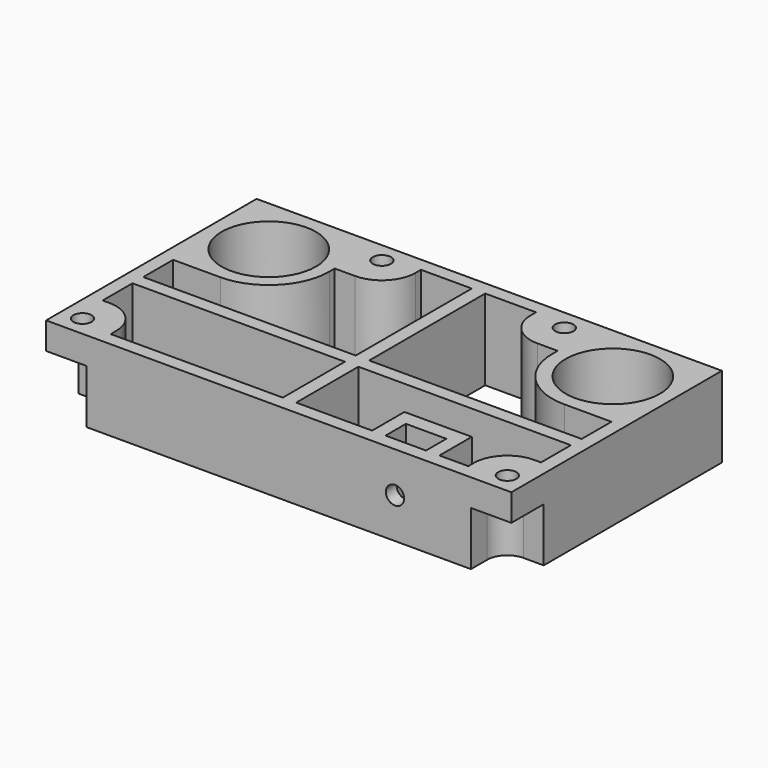
from build123d import *

# Parameters (mm, degrees)
F0_W      = 109.6809846
F0_H      = 62.036204
F0_R      = 2.15265
F0_W_2    = 9.525
F0_H_2    = 6
F0_R_2    = 11.1125
F1_DEPTH  = 19.05
F2_W      = 9.525
F2_H      = 9.525
F3_DEPTH  = 12.7
F4_R      = 4.76249
F6_DEPTH  = 19.05
F7_R      = 2.15265
F8_DEPTH  = 3.175
F9_R      = 1.7272
F10_DEPTH = 3.525


# Not quite as in the source:
# - a fillet or chamfer is up to 0.001 mm smaller than in the source, because OpenCascade refuses the exact size


with BuildPart() as f1:
    # F0 (on Top) → F1 (new body)
    with BuildSketch(Plane.XY):
        with Locations((0, -16.730602)):
            Rectangle(F0_W, F0_H)
        with Locations((-50.0779923, -42.986204)):
            Circle(F0_R, mode=Mode.SUBTRACT)
        with Locations((27.406219, -41.573704)):
            Rectangle(F0_W_2, F0_H_2, mode=Mode.SUBTRACT)
        with Locations((50.0779923, -42.986204)):
            Circle(F0_R, mode=Mode.SUBTRACT)
        with Locations((-40.5529923, 0)):
            Circle(F0_R_2, mode=Mode.SUBTRACT)
        with Locations((-21.5029923, 9.525)):
            Circle(F0_R, mode=Mode.SUBTRACT)
        with Locations((21.5029923, 9.525)):
            Circle(F0_R, mode=Mode.SUBTRACT)
        with Locations((40.5529923, 0)):
            Circle(F0_R_2, mode=Mode.SUBTRACT)
    extrude(amount=F1_DEPTH)

    # F2 (on face) → F3 (cut)
    with BuildSketch(Plane(origin=(0, 0, 0), x_dir=(1, 0, 0), z_dir=(0, 0, -1))):
        with Locations((-21.5029923, -9.525)):
            Rectangle(F2_W, F2_H)
        with Locations((21.5029923, -9.525)):
            Rectangle(F2_W, F2_H)
        with Locations((50.0779923, 42.986204)):
            Rectangle(F2_W, F2_H)
        with Locations((-50.0779923, 42.986204)):
            Rectangle(F2_W, F2_H)
    extrude(amount=-F3_DEPTH, mode=Mode.SUBTRACT)

    # F4 (radius 4.7625 in the source; OpenCascade refuses exactly that, so slightly less here)
    f4_edges = [f1.edges().sort_by_distance(p)[0] for p in [
        (-45.315492, -38.223704, 6.35),
        (45.315492, -38.223704, 6.35),
        (26.265492, 4.7625, 6.35),
        (16.740492, 4.7625, 6.35),
        (-26.265492, 4.7625, 6.35),
        (-16.740492, 4.7625, 6.35),
    ]]
    fillet(f4_edges, radius=F4_R)

    # F5 (on face) → F6 (cut, through all)
    with BuildSketch(Plane.XY.offset(19.05)):
        with BuildLine():
            Line((-51.6654923, -23.080602), (-1.5875, -23.080602))
            Line((-1.5875, -23.080602), (-1.5875, 11.1125))
            Line((-1.5875, 11.1125), (-13.5654923, 11.1125))
            Line((-13.5654923, 11.1125), (-13.5654923, 9.525))
            ThreePointArc((-13.5654923, 9.525), (-15.8903322243, 3.9123399243), (-21.5029923, 1.5875))
            Line((-21.5029923, 1.5875), (-26.2654923, 1.5875))
            Line((-26.2654923, 1.5875), (-26.2654923, 0))
            ThreePointArc((-26.2654923, 0), (-30.4502041638, -10.1027881362), (-40.5529923, -14.2875))
            Line((-40.5529923, -14.2875), (-51.6654923, -14.2875))
            Line((-51.6654923, -14.2875), (-51.6654923, -23.080602))
        make_face()
        with BuildLine():
            Line((-1.5875, -44.573704), (-1.5875, -26.255602))
            Line((-1.5875, -26.255602), (-51.6654923, -26.255602))
            Line((-51.6654923, -26.255602), (-51.6654923, -35.048704))
            Line((-51.6654923, -35.048704), (-50.0779923, -35.048704))
            ThreePointArc((-50.0779923, -35.048704), (-44.4653322243, -37.3735439243), (-42.1404923, -42.986204))
            Line((-42.1404923, -42.986204), (-42.1404923, -44.573704))
            Line((-42.1404923, -44.573704), (-1.5875, -44.573704))
        make_face()
        with BuildLine():
            Line((1.5875, -23.080602), (51.6654923, -23.080602))
            Line((51.6654923, -23.080602), (51.6654923, -14.2875))
            Line((51.6654923, -14.2875), (40.5529923, -14.2875))
            ThreePointArc((40.5529923, -14.2875), (30.4502041638, -10.1027881362), (26.2654923, 0))
            Line((26.2654923, 0), (26.2654923, 1.5875))
            Line((26.2654923, 1.5875), (21.5029923, 1.5875))
            ThreePointArc((21.5029923, 1.5875), (15.8903322243, 3.9123399243), (13.5654923, 9.525))
            Line((13.5654923, 9.525), (13.5654923, 11.1125))
            Line((13.5654923, 11.1125), (1.5875, 11.1125))
            Line((1.5875, 11.1125), (1.5875, -23.080602))
        make_face()
        with BuildLine():
            Line((51.6654923, -26.255602), (1.5875, -26.255602))
            Line((1.5875, -26.255602), (1.5875, -44.573704))
            Line((1.5875, -44.573704), (19.468719, -44.573704))
            Line((19.468719, -44.573704), (19.468719, -35.048704))
            Line((19.468719, -35.048704), (35.343719, -35.048704))
            Line((35.343719, -35.048704), (35.343719, -44.573704))
            Line((35.343719, -44.573704), (42.1404923, -44.573704))
            Line((42.1404923, -44.573704), (42.1404923, -42.986204))
            ThreePointArc((42.1404923, -42.986204), (44.4653322243, -37.3735439243), (50.0779923, -35.048704))
            Line((50.0779923, -35.048704), (51.6654923, -35.048704))
            Line((51.6654923, -35.048704), (51.6654923, -26.255602))
        make_face()
    extrude(amount=-F6_DEPTH, mode=Mode.SUBTRACT)

    # F7 (on face) → F8 (cut, through all)
    with BuildSketch(Plane.XZ.offset(47.748704)):
        with Locations((27.406219, 9.525)):
            Circle(F7_R)
    extrude(amount=-F8_DEPTH, mode=Mode.SUBTRACT)

    # F9 (on face) → F10 (cut, through all)
    with BuildSketch(Plane.XZ.offset(38.573704)):
        with Locations((27.406219, 9.525)):
            Circle(F9_R)
    extrude(amount=-F10_DEPTH, mode=Mode.SUBTRACT)


solid = f1.part
